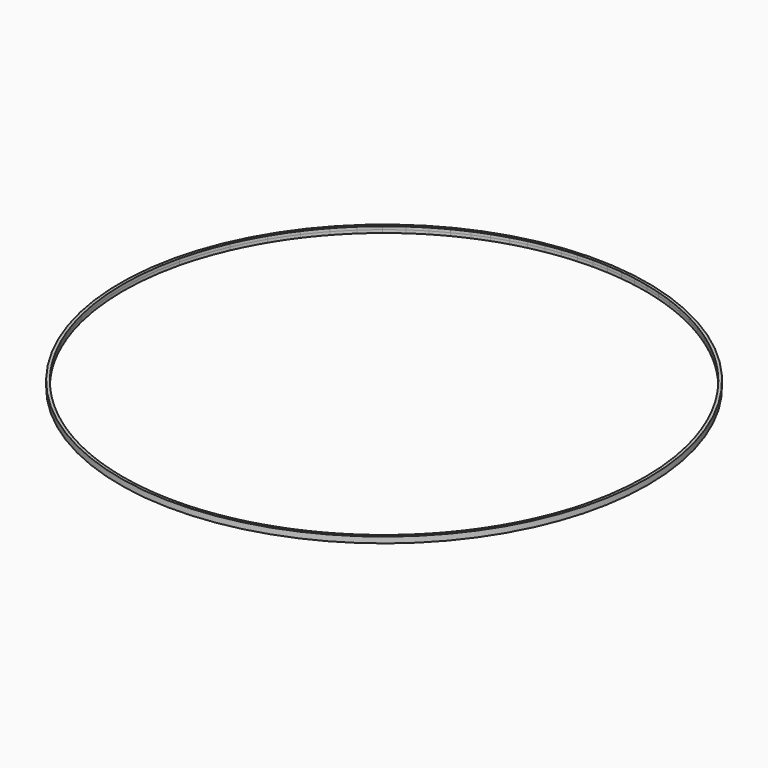
from build123d import *

# Parameters (mm, degrees)
F0_R     = 22.4700965803
F1_DEPTH = 0.254


# Not quite as in the source:
# - the program builds the solid bodies; features that only make, move or delete a surface that nothing else refers to are left out


with BuildPart() as f1:
    # F0 (on Top) → F1 (new body, symmetric)
    with BuildSketch(Plane.XY):
        Circle(F0_R)
        with BuildLine():
            ThreePointArc((21.5900000079, 5.2370647239), (22.0590171201, 2.6371785984), (22.2160965803, 0))
            ThreePointArc((22.2160965803, 0), (22.0590171201, -2.6371785984), (21.5900000079, -5.2370647239))
            ThreePointArc((21.5900000079, -5.2370647239), (21.0384334553, -7.1371748619), (20.3200000079, -8.9806763076))
            ThreePointArc((20.3200000079, -8.9806763076), (19.7230683789, -10.2252394097), (19.0500000079, -11.4303301336))
            ThreePointArc((19.0500000079, -11.4303301336), (18.4392268121, -12.3915237899), (17.7800000079, -13.3201556666))
            ThreePointArc((17.7800000079, -13.3201556666), (17.1623959089, -14.106988124), (16.5100000079, -14.8652227364))
            ThreePointArc((16.5100000079, -14.8652227364), (15.8882907181, -15.5279478787), (15.2400000079, -16.1646944612))
            ThreePointArc((15.2400000079, -16.1646944612), (14.6155298442, -16.7314444875), (13.9700000079, -17.2740859973))
            ThreePointArc((13.9700000079, -17.2740859973), (13.343529448, -17.7624651762), (12.7000000079, -18.2281361379))
            ThreePointArc((12.7000000079, -18.2281361379), (12.0719994886, -18.6499805794), (11.4300000079, -19.0501980852))
            ThreePointArc((11.4300000079, -19.0501980852), (10.8007791687, -19.413864031), (10.1600000079, -19.7567544679))
            ThreePointArc((10.1600000079, -19.7567544679), (9.5297718457, -20.0683431263), (8.8900000079, -20.3598341625))
            ThreePointArc((8.8900000079, -20.3598341625), (8.2589156398, -20.6239002063), (7.6200000079, -20.8684102687))
            ThreePointArc((7.6200000079, -20.8684102687), (6.9881687889, -21.0883959618), (6.3500000079, -21.2892566137))
            ThreePointArc((6.3500000079, -21.2892566137), (5.7175017639, -21.4677693495), (5.0800000079, -21.6274951667))
            ThreePointArc((5.0800000079, -21.6274951667), (4.4468927426, -21.7664901213), (3.8100000079, -21.8869560973))
            ThreePointArc((3.8100000079, -21.8869560973), (3.1763248591, -21.9878581871), (2.5400000079, -22.0704179214))
            ThreePointArc((2.5400000079, -22.0704179214), (1.9057844355, -22.1342027855), (1.2700000079, -22.1797666184))
            ThreePointArc((1.2700000079, -22.1797666184), (0.635259767, -22.2070122325), (0, -22.2160965803))
            ThreePointArc((0, -22.2160965803), (-0.635259767, -22.2070122325), (-1.2700000079, -22.1797666184))
            ThreePointArc((-1.2700000079, -22.1797666184), (-1.9057844355, -22.1342027855), (-2.5400000079, -22.0704179214))
            ThreePointArc((-2.5400000079, -22.0704179214), (-3.1763248591, -21.9878581871), (-3.8100000079, -21.8869560973))
            ThreePointArc((-3.8100000079, -21.8869560973), (-4.4468927426, -21.7664901213), (-5.0800000079, -21.6274951667))
            ThreePointArc((-5.0800000079, -21.6274951667), (-5.7175017639, -21.4677693495), (-6.3500000079, -21.2892566137))
            ThreePointArc((-6.3500000079, -21.2892566137), (-6.9881687889, -21.0883959618), (-7.6200000079, -20.8684102687))
            ThreePointArc((-7.6200000079, -20.8684102687), (-8.2589156398, -20.6239002063), (-8.8900000079, -20.3598341625))
            ThreePointArc((-8.8900000079, -20.3598341625), (-9.5297718457, -20.0683431263), (-10.1600000079, -19.7567544679))
            ThreePointArc((-10.1600000079, -19.7567544679), (-10.8007791687, -19.413864031), (-11.4300000079, -19.0501980852))
            ThreePointArc((-11.4300000079, -19.0501980852), (-12.0719994886, -18.6499805794), (-12.7000000079, -18.2281361379))
            ThreePointArc((-12.7000000079, -18.2281361379), (-13.343529448, -17.7624651762), (-13.9700000079, -17.2740859973))
            ThreePointArc((-13.9700000079, -17.2740859973), (-14.6155298442, -16.7314444875), (-15.2400000079, -16.1646944612))
            ThreePointArc((-15.2400000079, -16.1646944612), (-15.8882907181, -15.5279478787), (-16.5100000079, -14.8652227364))
            ThreePointArc((-16.5100000079, -14.8652227364), (-17.1623959089, -14.106988124), (-17.7800000079, -13.3201556666))
            ThreePointArc((-17.7800000079, -13.3201556666), (-18.4392268121, -12.3915237899), (-19.0500000079, -11.4303301336))
            ThreePointArc((-19.0500000079, -11.4303301336), (-19.7230683789, -10.2252394097), (-20.3200000079, -8.9806763076))
            ThreePointArc((-20.3200000079, -8.9806763076), (-21.0384334553, -7.1371748619), (-21.5900000079, -5.2370647239))
            ThreePointArc((-21.5900000079, -5.2370647239), (-22.2160965803, 0), (-21.5900000079, 5.2370647239))
            ThreePointArc((-21.5900000079, 5.2370647239), (-21.0384334553, 7.1371748619), (-20.3200000079, 8.9806763076))
            ThreePointArc((-20.3200000079, 8.9806763076), (-19.7230683789, 10.2252394097), (-19.0500000079, 11.4303301336))
            ThreePointArc((-19.0500000079, 11.4303301336), (-18.4392268121, 12.3915237899), (-17.7800000079, 13.3201556666))
            ThreePointArc((-17.7800000079, 13.3201556666), (-17.1623959089, 14.106988124), (-16.5100000079, 14.8652227364))
            ThreePointArc((-16.5100000079, 14.8652227364), (-15.8882907181, 15.5279478787), (-15.2400000079, 16.1646944612))
            ThreePointArc((-15.2400000079, 16.1646944612), (-14.6155298442, 16.7314444875), (-13.9700000079, 17.2740859973))
            ThreePointArc((-13.9700000079, 17.2740859973), (-13.343529448, 17.7624651762), (-12.7000000079, 18.2281361379))
            ThreePointArc((-12.7000000079, 18.2281361379), (-12.0719994886, 18.6499805794), (-11.4300000079, 19.0501980852))
            ThreePointArc((-11.4300000079, 19.0501980852), (-10.8007791687, 19.413864031), (-10.1600000079, 19.7567544679))
            ThreePointArc((-10.1600000079, 19.7567544679), (-9.5297718457, 20.0683431263), (-8.8900000079, 20.3598341625))
            ThreePointArc((-8.8900000079, 20.3598341625), (-8.2589156398, 20.6239002063), (-7.6200000079, 20.8684102687))
            ThreePointArc((-7.6200000079, 20.8684102687), (-6.9881687889, 21.0883959618), (-6.3500000079, 21.2892566137))
            ThreePointArc((-6.3500000079, 21.2892566137), (-5.7175017639, 21.4677693495), (-5.0800000079, 21.6274951667))
            ThreePointArc((-5.0800000079, 21.6274951667), (-4.4468927426, 21.7664901213), (-3.8100000079, 21.8869560973))
            ThreePointArc((-3.8100000079, 21.8869560973), (-3.1763248591, 21.9878581871), (-2.5400000079, 22.0704179214))
            ThreePointArc((-2.5400000079, 22.0704179214), (-1.9057844355, 22.1342027855), (-1.2700000079, 22.1797666184))
            ThreePointArc((-1.2700000079, 22.1797666184), (-0.635259767, 22.2070122325), (0, 22.2160965803))
            ThreePointArc((0, 22.2160965803), (0.635259767, 22.2070122325), (1.2700000079, 22.1797666184))
            ThreePointArc((1.2700000079, 22.1797666184), (1.9057844355, 22.1342027855), (2.5400000079, 22.0704179214))
            ThreePointArc((2.5400000079, 22.0704179214), (3.1763248591, 21.9878581871), (3.8100000079, 21.8869560973))
            ThreePointArc((3.8100000079, 21.8869560973), (4.4468927426, 21.7664901213), (5.0800000079, 21.6274951667))
            ThreePointArc((5.0800000079, 21.6274951667), (5.7175017639, 21.4677693495), (6.3500000079, 21.2892566137))
            ThreePointArc((6.3500000079, 21.2892566137), (6.9881687889, 21.0883959618), (7.6200000079, 20.8684102687))
            ThreePointArc((7.6200000079, 20.8684102687), (8.2589156398, 20.6239002063), (8.8900000079, 20.3598341625))
            ThreePointArc((8.8900000079, 20.3598341625), (9.5297718457, 20.0683431263), (10.1600000079, 19.7567544679))
            ThreePointArc((10.1600000079, 19.7567544679), (10.8007791687, 19.413864031), (11.4300000079, 19.0501980852))
            ThreePointArc((11.4300000079, 19.0501980852), (12.0719994886, 18.6499805794), (12.7000000079, 18.2281361379))
            ThreePointArc((12.7000000079, 18.2281361379), (13.343529448, 17.7624651762), (13.9700000079, 17.2740859973))
            ThreePointArc((13.9700000079, 17.2740859973), (14.6155298442, 16.7314444875), (15.2400000079, 16.1646944612))
            ThreePointArc((15.2400000079, 16.1646944612), (15.8882907181, 15.5279478787), (16.5100000079, 14.8652227364))
            ThreePointArc((16.5100000079, 14.8652227364), (17.1623959089, 14.106988124), (17.7800000079, 13.3201556666))
            ThreePointArc((17.7800000079, 13.3201556666), (18.4392268121, 12.3915237899), (19.0500000079, 11.4303301336))
            ThreePointArc((19.0500000079, 11.4303301336), (19.7230683789, 10.2252394097), (20.3200000079, 8.9806763076))
            ThreePointArc((20.3200000079, 8.9806763076), (21.0384334553, 7.1371748619), (21.5900000079, 5.2370647239))
        make_face(mode=Mode.SUBTRACT)
    extrude(amount=F1_DEPTH, both=True)


solid = f1.part
